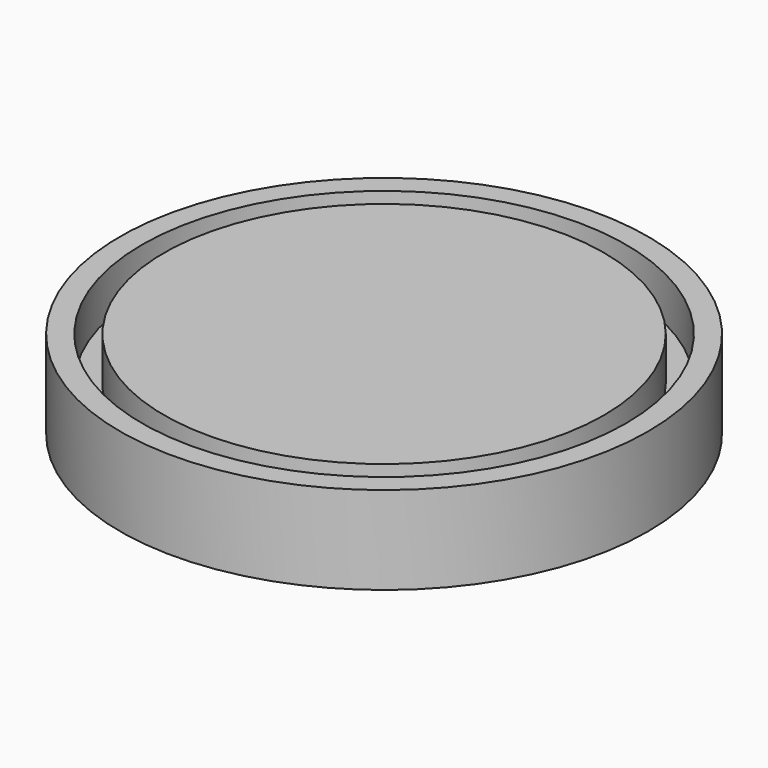
from build123d import *

# Parameters (mm, degrees)
F0_R      = 30
F0_R_2    = 27.5
F1_DEPTH  = 5
F2_DEPTH  = 10
F3_DEPTH  = 7.5
F4_R      = 30
F5_DEPTH  = 5
F6_R      = 30
F6_R_2    = 27.5
F7_DEPTH  = 2.5
F8_R      = 17.5
F9_DEPTH  = 3
F10_R     = 25
F11_DEPTH = 10


# Not quite as in the source:
# - a feature names something its author has since deleted; it is built from what else it names


with BuildPart() as f1:
    # F0 (on Top) → F1 (new body)
    with BuildSketch(Plane.XY):
        Circle(F0_R)
        Circle(F0_R_2, mode=Mode.SUBTRACT)
    extrude(amount=F1_DEPTH)

    # F0 (on Top) → F2 (join)
    with BuildSketch(Plane.XY):
        Circle(F0_R)
        Circle(F0_R_2, mode=Mode.SUBTRACT)
    extrude(amount=F2_DEPTH)

    # F0 (on Top) → F3 (join)
    with BuildSketch(Plane.XY):
        Circle(F0_R)
        Circle(F0_R_2, mode=Mode.SUBTRACT)
    extrude(amount=F3_DEPTH)

    # F4 (on Top) → F5 (join)
    with BuildSketch(Plane.XY):
        Circle(F4_R)
    extrude(amount=F5_DEPTH)

    # F6 (on Top) → F7 (join)
    with BuildSketch(Plane.XY):
        Circle(F6_R)
        Circle(F6_R_2, mode=Mode.SUBTRACT)
    extrude(amount=F7_DEPTH)

    # F8 (on Top) → F9 (join)
    with BuildSketch(Plane.XY):
        Circle(F8_R)
    extrude(amount=F9_DEPTH)

    # F10 (on Top) → F11 (join)
    with BuildSketch(Plane.XY):
        Circle(F10_R)
    extrude(amount=F11_DEPTH)


solid = f1.part
